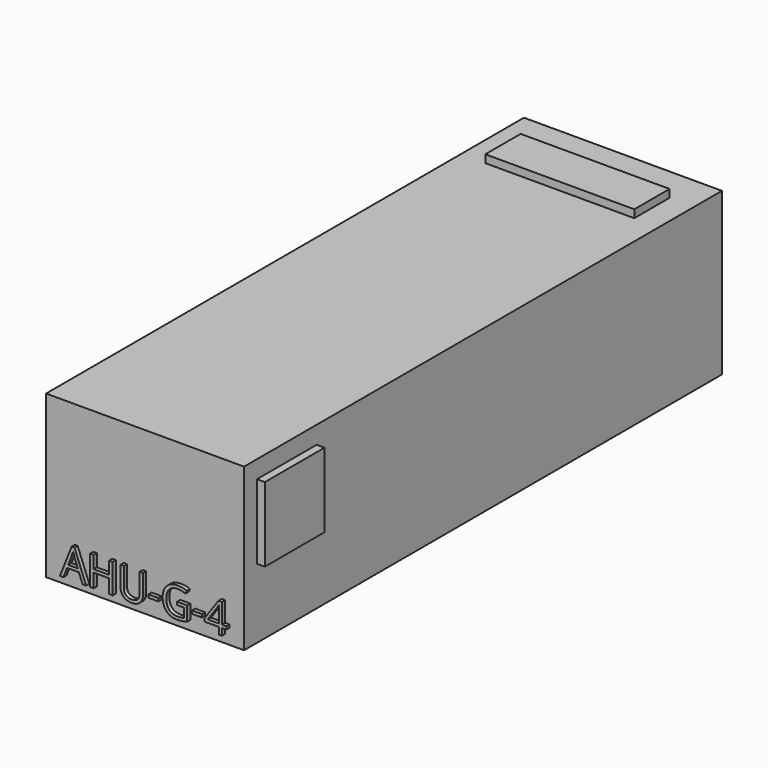
from build123d import *

# Parameters (mm, degrees)
F0_W         = 1282.7
F0_H         = 1047.75
F1_DEPTH     = 3870.325
F2_W         = 482.6
F2_H         = 482.6
F3_DEPTH     = 50.8
F4_TEXT_SIZE = 268.1662225061
F5_DEPTH     = 25.4
F6_W         = 965.2
F6_H         = 285.75
F7_DEPTH     = 50.8
F8_W         = 965.2
F8_H         = 285.75
F9_DEPTH     = 50.8
F10_W        = 685.8
F10_H        = 787.4
F10_W_2      = 254
F10_W_3      = 431.8
F11_DEPTH    = 6.35
F12_R        = 19.05
F12_R_2      = 25.4
F13_DEPTH    = 25.4


# Not quite as in the source:
# - Text() gives the source's letters only with a copy of the font that has no kerning and outlines rounded to 1/6400 em; it was checked with that copy


with BuildPart() as f1:
    # F0 (on Front) → F1 (new body)
    with BuildSketch(Plane.XZ):
        with Locations((1.4098696411, -28.5632179465)):
            Rectangle(F0_W, F0_H)
    extrude(amount=F1_DEPTH)

    # F2 (on face) → F3 (join)
    with BuildSketch(Plane.YZ.offset(642.7598696411)):
        with Locations((-3524.25, 139.7117820535)):
            Rectangle(F2_W, F2_H)
    extrude(amount=F3_DEPTH)

    # F4 (on face) → F5 (join)
    with BuildSketch(Plane.XZ.offset(3870.325)):
        with Locations((-529.784437269, -499.1856813431)):
            Text('AHU-G-4', F4_TEXT_SIZE, font='Open Sans', text_align=(TextAlign.LEFT, TextAlign.BOTTOM))
    extrude(amount=F5_DEPTH)

    # F6 (on face) → F7 (join)
    with BuildSketch(Plane.XY.offset(495.3117820535)):
        with Locations((1.4098696411, -368.3)):
            Rectangle(F6_W, F6_H)
    extrude(amount=F7_DEPTH)

    # F8 (on face) → F9 (join)
    with BuildSketch(Plane(origin=(0, 0, 0), x_dir=(-1, 0, 0), z_dir=(0, 1, 0))):
        with Locations((-1.4098696411, 50.8117820535)):
            Rectangle(F8_W, F8_H)
    extrude(amount=F9_DEPTH)

    # F10 (on face) → F11 (join)
    with BuildSketch(Plane(origin=(-639.9401303589, 0, 0), x_dir=(0, -1, 0), z_dir=(-1, 0, 0))):
        with Locations((415.925, 38.1117820535)):
            Rectangle(F10_W, F10_H)
        with Locations((987.425, 38.1117820535)):
            Rectangle(F10_W_2, F10_H)
        with Locations((1600.2, 38.1117820535)):
            Rectangle(F10_W_2, F10_H)
        with Locations((2444.75, 38.1117820535)):
            Rectangle(F10_W_2, F10_H)
        with Locations((3479.8, 38.1117820535)):
            Rectangle(F10_W_3, F10_H)
    extrude(amount=F11_DEPTH)

    # F12 (on face) → F13 (join)
    with BuildSketch(Plane(origin=(-639.9401303589, 0, 0), x_dir=(0, -1, 0), z_dir=(-1, 0, 0))):
        with Locations((1238.25, 114.3117820535)):
            Circle(F12_R)
        with Locations((1282.7, -76.1882179465)):
            Circle(F12_R)
        with Locations((1873.25, 57.1617820535)):
            Circle(F12_R_2)
        with Locations((2089.15, -19.0382179465)):
            Circle(F12_R_2)
    extrude(amount=F13_DEPTH)


solid = f1.part
